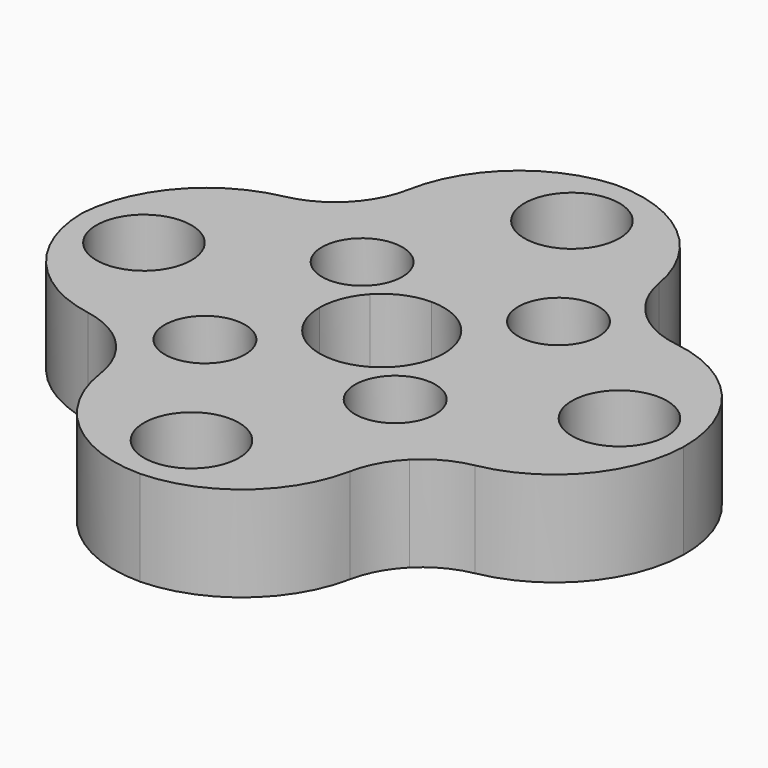
from build123d import *

# Parameters (mm, degrees)
F2_R        = 1.75
F3_DEPTH    = 6.5
F4_R        = 2.75
F5_DEPTH    = 3.5
F6_T1_DEPTH = 57.2838374918
F6_T3_DEPTH = 62.3332762367
F6_T5_DEPTH = 62.0777502529
F7_R        = 3.25
F8_DEPTH    = 4


# Not quite as in the source:
# - a fillet or chamfer that OpenCascade refuses, or shapes differently, is made with other operations: its cross-section is extruded or revolved along the edge and cut away or added


with BuildPart() as f3:
    # F2 (on Top) → F3 (new body)
    with BuildSketch(Plane.XY):
        with BuildLine():
            ThreePointArc((-3.1189043715, 2.8870288397), (-1.7018559621, 3.894378806), (0, 4.25))
            ThreePointArc((0, 4.25), (1.6264045876, 3.9264880132), (3.00520382, 3.00520382))
            Line((3.00520382, 3.00520382), (5.5861435714, 5.5861435714))
            ThreePointArc((5.5861435714, 5.5861435714), (5.5861435714, 7.8488852712), (7.8488852712, 7.8488852712))
            Line((7.8488852712, 7.8488852712), (10.0716416635, 10.0716416635))
            ThreePointArc((10.0716416635, 10.0716416635), (8.0706751581, 14.271751719), (9.6732808742, 18.6394108579))
            ThreePointArc((9.6732808742, 18.6394108579), (-0.2919239613, 20.9979708639), (-10.1877103957, 18.3632937376))
            ThreePointArc((-10.1877103957, 18.3632937376), (-9.2786875084, 16.6483019778), (-8.9647275629, 14.732852031))
            ThreePointArc((-8.9647275629, 14.732852031), (-9.4214503678, 12.4367514369), (-10.7220868758, 10.4902113439))
            Line((-10.7220868758, 10.4902113439), (-6.9029746628, 6.6710991309))
            ThreePointArc((-6.9029746628, 6.6710991309), (-5.1593103211, 7.017935533), (-4.1716038129, 5.539728281))
            ThreePointArc((-4.1716038129, 5.539728281), (-4.2933965608, 4.9274347892), (-4.640232963, 4.4083574311))
            Line((-4.640232963, 4.4083574311), (-3.1189043715, 2.8870288397))
        make_face()
        with BuildLine():
            ThreePointArc((0, 14.5134559673), (-1.2374368671, 17.5008928344), (1.75, 16.2634559673))
            ThreePointArc((1.75, 16.2634559673), (1.2374368671, 15.0260191002), (0, 14.5134559673))
        make_face(mode=Mode.SUBTRACT)
        with BuildLine():
            ThreePointArc((-4.25, 0), (-3.9571355536, 1.5503477708), (-3.1189043715, 2.8870288397))
            Line((-3.1189043715, 2.8870288397), (-4.640232963, 4.4083574311))
            ThreePointArc((-4.640232963, 4.4083574311), (-6.9029746628, 4.4083574311), (-6.9029746628, 6.6710991309))
            Line((-6.9029746628, 6.6710991309), (-10.7220868758, 10.4902113439))
            ThreePointArc((-10.7220868758, 10.4902113439), (-14.5116932272, 8.7499798202), (-18.5201343168, 9.899728526))
            ThreePointArc((-18.5201343168, 9.899728526), (-20.9996146914, 0.1272116798), (-18.6387120488, -9.674627288))
            ThreePointArc((-18.6387120488, -9.674627288), (-14.279821029, -8.0983145468), (-10.0983841523, -10.0983841523))
            Line((-10.0983841523, -10.0983841523), (-7.8488852712, -7.8488852712))
            ThreePointArc((-7.8488852712, -7.8488852712), (-7.8488852712, -5.5861435714), (-5.5861435714, -5.5861435714))
            Line((-5.5861435714, -5.5861435714), (-3.00520382, -3.00520382))
            ThreePointArc((-3.00520382, -3.00520382), (-3.9264880132, -1.6264045876), (-4.25, 0))
        make_face()
        with Locations((-16.2634559673, 0)):
            Circle(F2_R, mode=Mode.SUBTRACT)
        with BuildLine():
            Line((5.5861435714, 5.5861435714), (3.00520382, 3.00520382))
            ThreePointArc((3.00520382, 3.00520382), (3.9264880132, 1.6264045876), (4.25, 0))
            ThreePointArc((4.25, 0), (3.894378806, -1.7018559621), (2.8870288397, -3.1189043715))
            Line((2.8870288397, -3.1189043715), (4.4083574311, -4.640232963))
            ThreePointArc((4.4083574311, -4.640232963), (6.1520217728, -4.2933965608), (7.139728281, -5.7716038129))
            ThreePointArc((7.139728281, -5.7716038129), (7.017935533, -6.3838973046), (6.6710991309, -6.9029746628))
            Line((6.6710991309, -6.9029746628), (10.4902113439, -10.7220868758))
            ThreePointArc((10.4902113439, -10.7220868758), (14.3265437078, -8.9785005753), (18.3632937376, -10.1877103957))
            ThreePointArc((18.3632937376, -10.1877103957), (20.3301397989, -5.2616932403), (21, 0))
            ThreePointArc((21, 0), (20.3137902, 5.3244650163), (18.3000068848, 10.3009585969))
            ThreePointArc((18.3000068848, 10.3009585969), (14.2313497781, 8.552751018), (10.0716416635, 10.0716416635))
            Line((10.0716416635, 10.0716416635), (7.8488852712, 7.8488852712))
            ThreePointArc((7.8488852712, 7.8488852712), (8.1957216733, 7.3298079131), (8.3175144213, 6.7175144213))
            ThreePointArc((8.3175144213, 6.7175144213), (7.3298079131, 5.2393071693), (5.5861435714, 5.5861435714))
        make_face()
        with BuildLine():
            ThreePointArc((18.0134559673, 0), (16.2634559673, -1.75), (14.5134559673, 0))
            ThreePointArc((14.5134559673, 0), (16.2634559673, 1.75), (18.0134559673, 0))
        make_face(mode=Mode.SUBTRACT)
        with BuildLine():
            Line((4.4083574311, -4.640232963), (2.8870288397, -3.1189043715))
            ThreePointArc((2.8870288397, -3.1189043715), (1.5503477708, -3.9571355536), (0, -4.25))
            ThreePointArc((0, -4.25), (-1.6264045876, -3.9264880132), (-3.00520382, -3.00520382))
            Line((-3.00520382, -3.00520382), (-5.5861435714, -5.5861435714))
            ThreePointArc((-5.5861435714, -5.5861435714), (-5.2393071693, -6.1052209295), (-5.1175144213, -6.7175144213))
            ThreePointArc((-5.1175144213, -6.7175144213), (-6.1052209295, -8.1957216733), (-7.8488852712, -7.8488852712))
            Line((-7.8488852712, -7.8488852712), (-10.0983841523, -10.0983841523))
            ThreePointArc((-10.0983841523, -10.0983841523), (-8.9703530251, -11.9546705323), (-8.577165246, -14.0909422189))
            ThreePointArc((-8.577165246, -14.0909422189), (-9.024856678, -16.365116699), (-10.301121768, -18.2999150359))
            ThreePointArc((-10.301121768, -18.2999150359), (-0.2289175978, -20.9987522661), (9.899728526, -18.5201343168))
            ThreePointArc((9.899728526, -18.5201343168), (8.7499798202, -14.5116932272), (10.4902113439, -10.7220868758))
            Line((10.4902113439, -10.7220868758), (6.6710991309, -6.9029746628))
            ThreePointArc((6.6710991309, -6.9029746628), (4.4083574311, -6.9029746628), (4.4083574311, -4.640232963))
        make_face()
        with BuildLine():
            ThreePointArc((1.75, -16.2634559673), (-1.2374368671, -17.5008928344), (0, -14.5134559673))
            ThreePointArc((0, -14.5134559673), (1.2374368671, -15.0260191002), (1.75, -16.2634559673))
        make_face(mode=Mode.SUBTRACT)
    extrude(amount=F3_DEPTH)

    # F4 (on face) → F5 (cut)
    with BuildSketch(Plane.XY.offset(6.5)):
        with Locations((-5.7716038129, 5.539728281)):
            Circle(F4_R)
        with Locations((5.539728281, -5.7716038129)):
            Circle(F4_R)
        with Locations((-6.7175144213, -6.7175144213)):
            Circle(F4_R)
        with Locations((6.7175144213, 6.7175144213)):
            Circle(F4_R)
    extrude(amount=-F5_DEPTH, mode=Mode.SUBTRACT)

    # F6: fillet of radius 9 on 8 edges, made by hand

    # F6_s2 → F6_t1 (cut)
    with BuildSketch(Plane.XY.offset(-25.3919187459)):
        with BuildLine():
            ThreePointArc((-0.3782425644, 20.9965933561), (-6.0328802021, 18.8657689221), (-9.065291981, 13.6389325572))
            ThreePointArc((-9.065291981, 13.6389325572), (-9.1272145679, 16.1197341578), (-10.1877103957, 18.3632937376))
            ThreePointArc((-10.1877103957, 18.3632937376), (-5.4445759439, 20.2819277385), (-0.3782425644, 20.9965933561))
        make_face()
        with BuildLine():
            ThreePointArc((20.9965933561, -0.3782425644), (18.8657689221, -6.0328802021), (13.6389325572, -9.065291981))
            ThreePointArc((13.6389325572, -9.065291981), (16.1197341578, -9.1272145679), (18.3632937376, -10.1877103957))
            ThreePointArc((18.3632937376, -10.1877103957), (20.2819277385, -5.4445759439), (20.9965933561, -0.3782425644))
        make_face()
        with BuildLine():
            ThreePointArc((-13.7788227476, 8.8512170739), (-18.9576712537, 5.7375588181), (-20.9999396683, 0.0503381168))
            ThreePointArc((-20.9999396683, 0.0503381168), (-20.3644711398, 5.1272131997), (-18.5201343168, 9.899728526))
            ThreePointArc((-18.5201343168, 9.899728526), (-16.2602888025, 8.8743948046), (-13.7788227476, 8.8512170739))
        make_face()
        with BuildLine():
            ThreePointArc((0.0503381168, -20.9999396683), (5.7375588181, -18.9576712537), (8.8512170739, -13.7788227476))
            ThreePointArc((8.8512170739, -13.7788227476), (8.8743948046, -16.2602888025), (9.899728526, -18.5201343168))
            ThreePointArc((9.899728526, -18.5201343168), (5.1272131997, -20.3644711398), (0.0503381168, -20.9999396683))
        make_face()
    extrude(amount=F6_T1_DEPTH, mode=Mode.SUBTRACT)

    # F6_s4 → F6_t3 (cut)
    with BuildSketch(Plane.XY.offset(-27.9166381183)):
        with BuildLine():
            ThreePointArc((-1.2489870314, 20.962824986), (4.8716041748, 19.0359733336), (8.1530373835, 13.5217562449))
            ThreePointArc((8.1530373835, 13.5217562449), (8.3126072664, 16.2589826676), (9.6732808742, 18.6394108579))
            ThreePointArc((9.6732808742, 18.6394108579), (4.3694101421, 20.5404054247), (-1.2489870314, 20.962824986))
        make_face()
        with BuildLine():
            ThreePointArc((13.2369559696, 8.6077236934), (18.8594743215, 5.515526839), (20.993156783, -0.5360674268))
            ThreePointArc((20.993156783, -0.5360674268), (20.3800996321, 5.0647348385), (18.3000068848, 10.3009585969))
            ThreePointArc((18.3000068848, 10.3009585969), (15.9671809198, 8.8601969743), (13.2369559696, 8.6077236934))
        make_face()
    extrude(amount=F6_T3_DEPTH, mode=Mode.SUBTRACT)

    # F6_s6 → F6_t5 (cut)
    with BuildSketch(Plane.XY.offset(-27.7888751265)):
        with BuildLine():
            ThreePointArc((-8.6359238746, -13.2532961322), (-5.5485972344, -18.85793385), (0.4828918194, -20.9944472538))
            ThreePointArc((0.4828918194, -20.9944472538), (-5.090632161, -20.3736463158), (-10.301121768, -18.2999150359))
            ThreePointArc((-10.301121768, -18.2999150359), (-8.8793307439, -15.9710172139), (-8.6359238746, -13.2532961322))
        make_face()
        with BuildLine():
            ThreePointArc((-20.9659970002, 1.1945584074), (-19.0352466943, -4.9059131307), (-13.5385270334, -8.1815234096))
            ThreePointArc((-13.5385270334, -8.1815234096), (-16.2629392178, -8.3326294351), (-18.6387120488, -9.674627288))
            ThreePointArc((-18.6387120488, -9.674627288), (-20.5345573153, -4.3968120117), (-20.9659970002, 1.1945584074))
        make_face()
    extrude(amount=F6_T5_DEPTH, mode=Mode.SUBTRACT)

    # F7 (on face) → F8 (cut)
    with BuildSketch(Plane.XY.offset(6.5)):
        with Locations((-16.2634559673, 0)):
            Circle(F7_R)
        with Locations((0, 16.2634559673)):
            Circle(F7_R)
        with Locations((16.2634559673, 0)):
            Circle(F7_R)
        with Locations((0, -16.2634559673)):
            Circle(F7_R)
    extrude(amount=-F8_DEPTH, mode=Mode.SUBTRACT)


solid = f3.part
